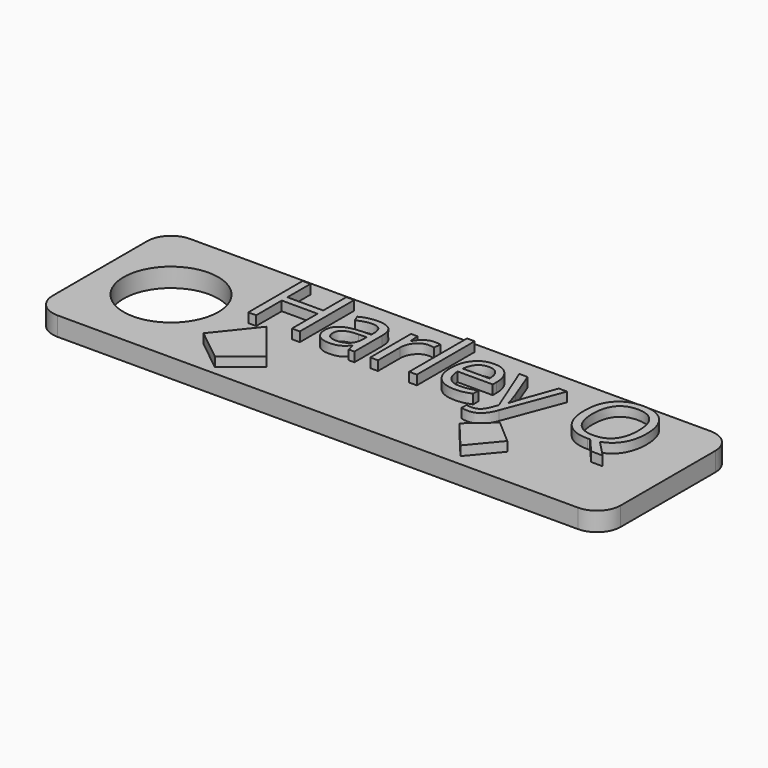
from build123d import *

# Parameters (mm, degrees)
F0_W         = 120
F0_H         = 35
F0_R         = 10
F1_DEPTH     = 4
F2_R         = 5
F3_TEXT_SIZE = 20.1117350823
F5_DEPTH     = 2
F6_DEPTH     = 2


# Not quite as in the source:
# - Text() gives the source's letters only with a copy of the font that has no kerning and outlines rounded to 1/6400 em; it was checked with that copy


with BuildPart() as f1:
    # F0 (on Top) → F1 (new body)
    with BuildSketch(Plane.XY):
        Rectangle(F0_W, F0_H)
        with Locations((-45, 0)):
            Circle(F0_R, mode=Mode.SUBTRACT)
    extrude(amount=F1_DEPTH)

    # F2
    f2_edges = [f1.edges().sort_by_distance(p)[0] for p in [
        (60, 17.5, 2),
        (60, -17.5, 2),
        (-60, -17.5, 2),
        (-60, 17.5, 2),
    ]]
    fillet(f2_edges, radius=F2_R)

    # F3 (on face) → F5 (join)
    with BuildSketch(Plane.XY.offset(4)):
        with Locations((-30.6526676422, 0)):
            Text('Harley Q', F3_TEXT_SIZE, font='Open Sans', text_align=(TextAlign.LEFT, TextAlign.BOTTOM))
    extrude(amount=F5_DEPTH)

    # F4 (on face) → F6 (join)
    with BuildSketch(Plane.XY.offset(4)):
        Polygon((-23.1319088489, -15.7555118203), (-16.4841556537, -10.4373112268), (-23.1319088489, -2.1276166663), (-29.7796620441, -10.4373112268), align=None)
        Polygon((33.3985071629, -9.1939466074), (28.3511448652, -4.8107143332), (23.3037825674, -9.1939466074), (28.3511448652, -15.2507759631), align=None)
    extrude(amount=F6_DEPTH)


solid = f1.part
